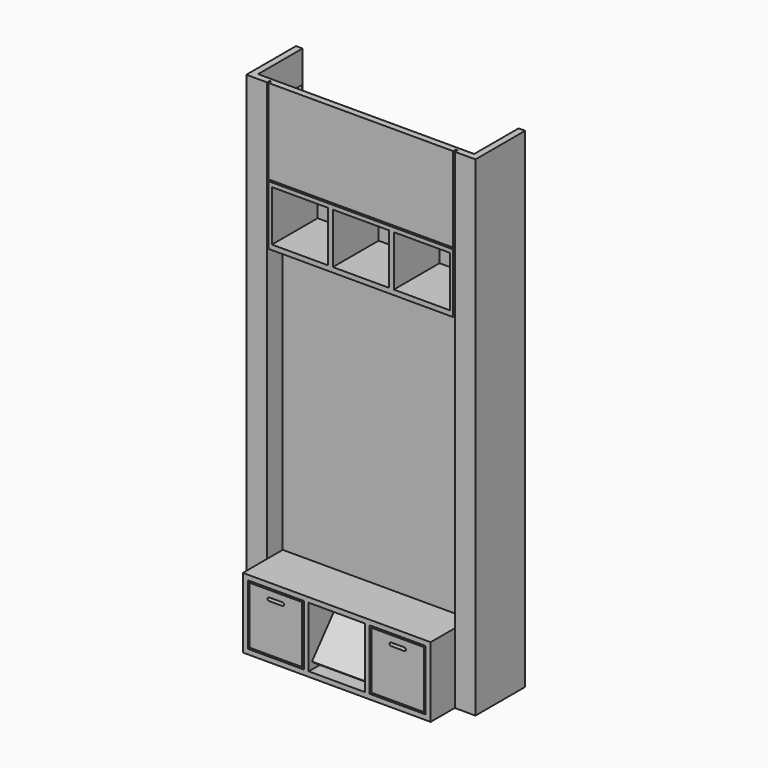
from build123d import *

# Parameters (mm, degrees)
F0_W           = 57.5
F0_H           = 21.5
F0_W_2         = 17.1666666667
F0_H_2         = 18.5
F1_DEPTH       = 16.75
F2_W           = 17.1666666667
F2_H           = 18.5
F3_DEPTH       = 2
F4_W           = 17.1666666667
F4_H           = 18.5
F4_W_2         = 16.1666666667
F4_H_2         = 17.5
F5_DEPTH       = 1
F7_DEPTH       = 16.751
F9_DEPTH       = 17.1666666667
F10_W          = 57.5
F10_H          = 1.5
F11_DEPTH      = 83.75
F13_W          = 57.5
F13_H          = 18.5
F14_DEPTH      = 19
F15_W          = 17.1666666667
F15_H          = 15.5
F16_DEPTH      = 17.5
F17_W          = 2
F17_H          = 26.25
F18_DEPTH      = 28.75
F18_DEPTH_BACK = 28.75
F20_DEPTH      = 150
F21_W          = 1
F21_H          = 5.5
F22_DEPTH      = 106.2
F24_DEPTH      = 1
F27_DEPTH      = 1.5
F30_DEPTH      = 1.5


# Not quite as in the source:
# - a pattern or mirror of a feature is missing from the dataset's text; its kind, count and spacing are read off the source's solid


with BuildPart() as f1:
    # F0 (on Front) → F1 (new body)
    with BuildSketch(Plane.XZ):
        with Locations((0, 10.75)):
            Rectangle(F0_W, F0_H)
        with Locations((-18.6666666667, 10.75)):
            Rectangle(F0_W_2, F0_H_2, mode=Mode.SUBTRACT)
        with Locations((0, 10.75)):
            Rectangle(F0_W_2, F0_H_2, mode=Mode.SUBTRACT)
        with Locations((18.6666666667, 10.75)):
            Rectangle(F0_W_2, F0_H_2, mode=Mode.SUBTRACT)
    extrude(amount=F1_DEPTH)

    # F2 (on face) → F3 (join)
    with BuildSketch(Plane.XZ.offset(16.75)):
        with Locations((-18.6666666667, 10.75)):
            Rectangle(F2_W, F2_H)
        with Locations((18.6666666667, 10.75)):
            Rectangle(F2_W, F2_H)
    extrude(amount=-F3_DEPTH)

    # F4 (on face) → F5 (cut)
    with BuildSketch(Plane.XZ.offset(16.75)):
        with Locations((-18.6666666667, 10.75)):
            Rectangle(F4_W, F4_H)
        with Locations((-18.6666666667, 10.75)):
            Rectangle(F4_W_2, F4_H_2, mode=Mode.SUBTRACT)
    f5 = extrude(amount=-F5_DEPTH, mode=Mode.SUBTRACT)

    # F5_copies: F5 across plane
    add(f5.mirror(Plane(origin=(0, 0, 0), x_dir=(0, 0, 1), z_dir=(1, 0, 0))), mode=Mode.SUBTRACT)

    # F6 (on face) → F7 (cut, through all)
    with BuildSketch(Plane.XZ.offset(16.75)):
        with BuildLine():
            Line((-16.6666666667, 17.5), (-20.6666666667, 17.5))
            ThreePointArc((-20.6666666667, 17.5), (-21.0202200573, 17.3535533906), (-21.1666666667, 17))
            ThreePointArc((-21.1666666667, 17), (-21.0202200573, 16.6464466094), (-20.6666666667, 16.5))
            Line((-20.6666666667, 16.5), (-16.6666666667, 16.5))
            ThreePointArc((-16.6666666667, 16.5), (-16.3131132761, 16.6464466094), (-16.1666666667, 17))
            ThreePointArc((-16.1666666667, 17), (-16.3131132761, 17.3535533906), (-16.6666666667, 17.5))
        make_face()
    f7 = extrude(amount=-F7_DEPTH, mode=Mode.SUBTRACT)

    # F7_copies: F7 across plane
    add(f7.mirror(Plane(origin=(0, 0, 0), x_dir=(0, 0, 1), z_dir=(1, 0, 0))), mode=Mode.SUBTRACT)

    # F8 (on face) → F9 (join, through all)
    with BuildSketch(Plane.YZ.offset(-8.5833333333)):
        Polygon((-15.5160444431, 3.6427876097), (-14.75, 3), (-4.465398245, 15.2567110899), (-5.2314426881, 15.8994986996), align=None)
    extrude(amount=F9_DEPTH)

    # F10 (on face) → F11 (join)
    with BuildSketch(Plane.XY.offset(21.5)):
        with Locations((0, -0.75)):
            Rectangle(F10_W, F10_H)
    extrude(amount=F11_DEPTH)

    # F13 (on offset) → F14 (join)
    with BuildSketch(Plane.XZ.offset(7.5)):
        with Locations((0, 114.5)):
            Rectangle(F13_W, F13_H)
    extrude(amount=-F14_DEPTH)

    # F15 (on face) → F16 (cut)
    with BuildSketch(Plane.XZ.offset(7.5)):
        with Locations((-18.6666666667, 114.5)):
            Rectangle(F15_W, F15_H)
        with Locations((0, 114.5)):
            Rectangle(F15_W, F15_H)
        with Locations((18.6666666667, 114.5)):
            Rectangle(F15_W, F15_H)
    extrude(amount=-F16_DEPTH, mode=Mode.SUBTRACT)

    # F17 (on Right) → F18 (join, two sides)
    with BuildSketch(Plane.YZ) as f18_sk:
        with Locations((-6.5, 136.875)):
            Rectangle(F17_W, F17_H)
    extrude(amount=F18_DEPTH)
    extrude(f18_sk.sketch, amount=-F18_DEPTH_BACK)

    # F19 (on Top) → F20 (join, through all)
    with BuildSketch(Plane.XY):
        Polygon((-35.0999999999, -7.5), (-28.7499999999, -7.5), (-28.7499999999, -5.5), (-33.0999999999, -5.5), (-33.0999999999, 11.5), (-35.0999999999, 11.5), align=None)
        Polygon((35.0999999999, -7.5), (35.0999999999, 11.5), (33.0999999999, 11.5), (33.0999999999, -5.5), (28.7499999999, -5.5), (28.7499999999, -7.5), align=None)
    extrude(amount=F20_DEPTH)

    # F21 (on Top) → F22 (join)
    with BuildSketch(Plane.XY):
        with Locations((-29.2499999999, -2.75)):
            Rectangle(F21_W, F21_H)
        with Locations((29.2499999999, -2.75)):
            Rectangle(F21_W, F21_H)
    extrude(amount=F22_DEPTH)

    # F23 (on face) → F24 (cut)
    with BuildSketch(Plane.XZ.offset(7.5)):
        Polygon((28.2499999999, 105.2500000002), (28.7499999999, 105.2500000002), (28.7499999999, 150), (28.2499999999, 150), (28.2499999999, 124), (-28.25, 124), (-28.2499999999, 150), (-28.7499999999, 150), (-28.7499999999, 105.2500000002), (-28.2499999999, 105.2500000002), (-28.2499999999, 123.5), (28.25, 123.5), align=None)
    extrude(amount=-F24_DEPTH, mode=Mode.SUBTRACT)

    # F26 (on offset) → F27 (join)
    with BuildSketch(Plane.XY.offset(138.75)):
        Polygon((-21.0999999999, -5.5), (-33.0999999999, 11.5), (-33.0999999999, -5.5), align=None)
    f27 = extrude(amount=F27_DEPTH)

    # F27_copies: F27 across plane
    add(f27.mirror(Plane(origin=(0, 0, 0), x_dir=(0, 0, 1), z_dir=(1, 0, 0))))

    # F29 (on offset) → F30 (join)
    with BuildSketch(Plane.XY.offset(25)):
        Polygon((-33.0999999999, 4.7458333333), (-29.7499999999, 0), (-24.9823529411, 0), (-33.0999999999, 11.5), align=None)
    f30 = extrude(amount=F30_DEPTH)

    # F30_copies: F30 across plane
    add(f30.mirror(Plane(origin=(0, 0, 0), x_dir=(0, 0, 1), z_dir=(1, 0, 0))))


solid = f1.part
